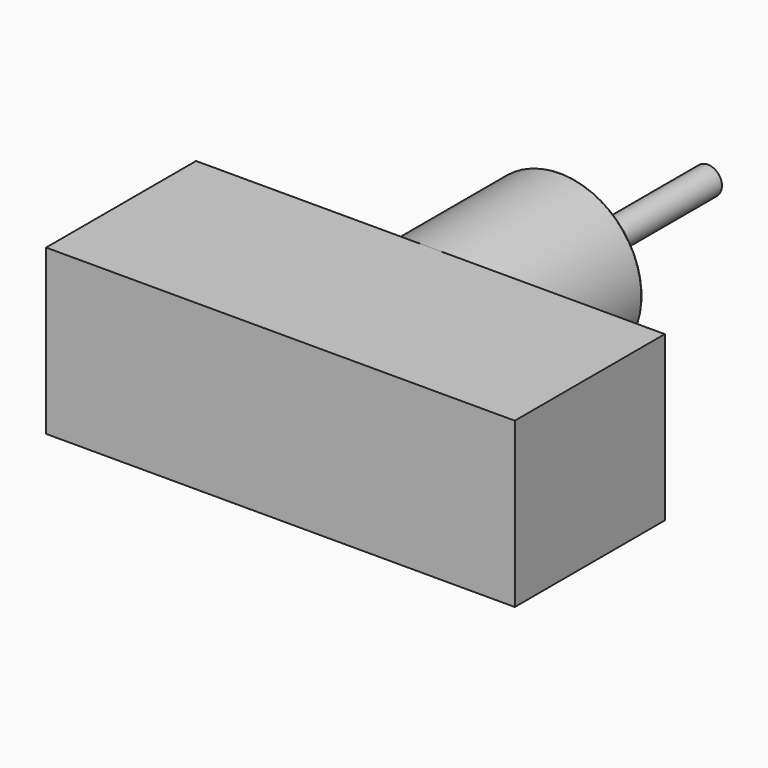
from build123d import *

# Parameters (mm, degrees)
F2_R     = 2
F4_DEPTH = 20


with BuildPart() as f1:
    # F0 (on Top) → F1 (revolve)
    with BuildSketch(Plane.XY):
        with BuildLine():
            Line((-8.75, 0), (0, 0))
            Line((0, 0), (0, 37))
            Line((0, 37), (-1.5, 37))
            Line((-1.5, 37), (-1.5, 15.3282299509))
            ThreePointArc((-1.5, 15.3282299509), (-4.3322917664, 13.3172311391), (-7.1645835327, 15.3282299509))
            Line((-7.1645835327, 15.3282299509), (-7.8059027445, 17.1648335314))
            ThreePointArc((-7.8059027445, 17.1648335314), (-8.2779513723, 17.5), (-8.75, 17.1648335314))
            Line((-8.75, 17.1648335314), (-8.75, 0))
        make_face()
    revolve(axis=Axis((0, 18.5, 0), (0, -1, 0)))

    # F2
    f2_edges = [f1.edges().sort_by_distance(p)[0] for p in [
        (1.5, 15.32823, 0),
    ]]
    fillet(f2_edges, radius=F2_R)

    # F3 (on face) → F4 (join)
    with BuildSketch(Plane.XZ):
        with BuildLine():
            Line((9.5e-09, 8.75), (-25, 8.75))
            Line((-25, 8.75), (-25, -8.75))
            Line((-25, -8.75), (0, -8.75))
            ThreePointArc((0, -8.75), (-8.75, 4.8e-09), (9.5e-09, 8.75))
        make_face()
        with BuildLine():
            Line((25, 8.75), (9.5e-09, 8.75))
            ThreePointArc((9.5e-09, 8.75), (6.1871843388, 6.187184332), (8.75, 0))
            ThreePointArc((8.75, 0), (6.1871843354, -6.1871843354), (0, -8.75))
            Line((0, -8.75), (25, -8.75))
            Line((25, -8.75), (25, 8.75))
        make_face()
        with BuildLine():
            ThreePointArc((8.75, 0), (6.1871843388, 6.187184332), (9.5e-09, 8.75))
            ThreePointArc((9.5e-09, 8.75), (-8.75, 4.8e-09), (0, -8.75))
            ThreePointArc((0, -8.75), (6.1871843354, -6.1871843354), (8.75, 0))
        make_face()
    extrude(amount=F4_DEPTH)


solid = f1.part
